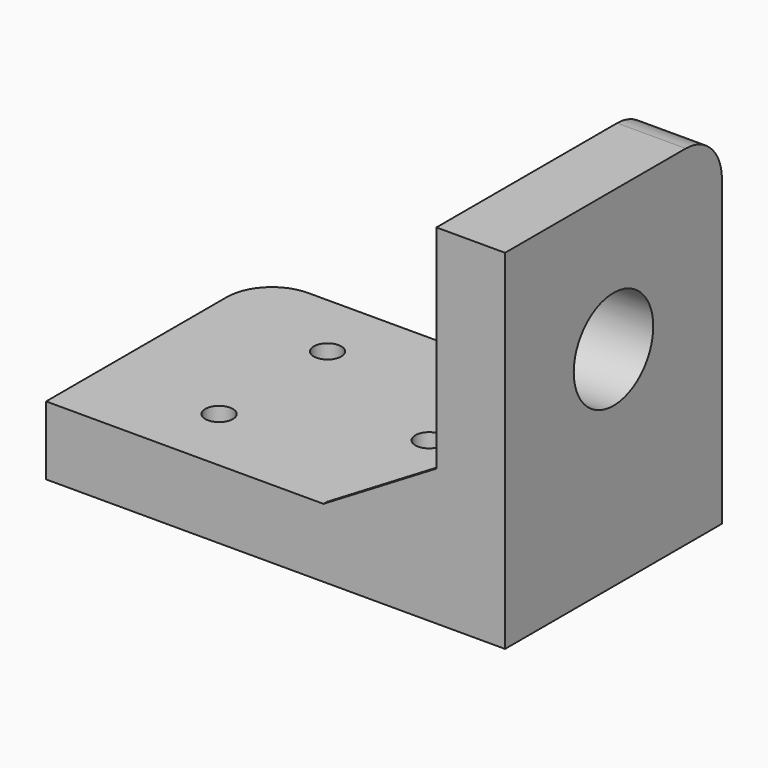
from build123d import *

# Parameters (mm, degrees)
F0_W          = 50.8
F0_H          = 30
F0_R          = 1.525
F1_DEPTH      = 7.6
F2_W          = 7.6
F2_H          = 30
F3_DEPTH      = 31
F4_R          = 5.5
F5_DEPTH      = 7.6
F6_R          = 5
F9_DEPTH      = 7
F10_DEPTH     = 7
F11_T4_DEPTH  = 48.0092585807
F11_T10_DEPTH = 48.0092585807


# Not quite as in the source:
# - a fillet or chamfer that OpenCascade refuses, or shapes differently, is made with other operations: its cross-section is extruded or revolved along the edge and cut away or added


with BuildPart() as f1:
    # F0 (on Top) → F1 (new body)
    with BuildSketch(Plane.XY):
        Rectangle(F0_W, F0_H)
        with Locations((-12.25, -7.5)):
            Circle(F0_R, mode=Mode.SUBTRACT)
        with Locations((-12.25, 7.5)):
            Circle(F0_R, mode=Mode.SUBTRACT)
        with Locations((5, 0)):
            Circle(F0_R, mode=Mode.SUBTRACT)
    extrude(amount=F1_DEPTH)

    # F2 (on face) → F3 (join)
    with BuildSketch(Plane.XY.offset(7.6)):
        with Locations((21.6, 0)):
            Rectangle(F2_W, F2_H)
    extrude(amount=F3_DEPTH)

    # F4 (on face) → F5 (cut)
    with BuildSketch(Plane(origin=(17.8, 0, 0), x_dir=(0, -1, 0), z_dir=(-1, 0, 0))):
        with Locations((0, 23.1)):
            Circle(F4_R)
    extrude(amount=-F5_DEPTH, mode=Mode.SUBTRACT)

    # F6
    f6_edges = [f1.edges().sort_by_distance(p)[0] for p in [
        (21.6, 15, 38.6),
        (-25.4, 15, 3.8),
    ]]
    fillet(f6_edges, radius=F6_R)

    # F7 (on face) → F9 (join)
    with BuildSketch(Plane(origin=(0, 15, 0), x_dir=(-1, 0, 0), z_dir=(0, 1, 0))):
        Polygon((-5.3, 7.6), (-17.8, 15.1), (-17.8, 7.6), align=None)
    extrude(amount=-F9_DEPTH)

    # F8 (on face) → F10 (join)
    with BuildSketch(Plane.XZ.offset(15)):
        Polygon((17.8, 7.6), (17.8, 15.1), (5.3, 7.6), align=None)
    extrude(amount=-F10_DEPTH)

    # F11: chamfer of 6.5 on 2 edges, made by hand


with BuildPart() as f11_tool2:
    # F11_s3 → F11_t4 (new body)
    with BuildSketch(Plane(origin=(-7.0837998008, 0, -4.2502798805), x_dir=(0, 1, 0), z_dir=(0.8574929257, 0, 0.5144957554))):
        Polygon((14.5, 3.7901187316), (8, -2.7098812684), (8, 3.7901187316), align=None)
    extrude(amount=F11_T4_DEPTH)

    split(bisect_by=Plane.YZ.offset(17.8), keep=Keep.BOTTOM)

    split(bisect_by=Plane.XY.offset(7.6), keep=Keep.TOP)


with BuildPart() as f1_1:
    add(f1.part)

    # F11_t1: cut F11_tool2
    add(f11_tool2.part, mode=Mode.SUBTRACT)


with BuildPart() as f11_tool8:
    # F11_s9 → F11_t10 (new body)
    with BuildSketch(Plane(origin=(34.0837998008, 0, 20.4502798805), x_dir=(0, 1, 0), z_dir=(-0.8574929257, 0, -0.5144957554))):
        Polygon((-8, 2.7098812684), (-14.5, -3.7901187316), (-8, -3.7901187316), align=None)
    extrude(amount=F11_T10_DEPTH)

    split(bisect_by=Plane.YZ.offset(17.8), keep=Keep.BOTTOM)

    split(bisect_by=Plane.XY.offset(7.6), keep=Keep.TOP)


with BuildPart() as f1_2:
    add(f1_1.part)

    # F11_t7: cut F11_tool8
    add(f11_tool8.part, mode=Mode.SUBTRACT)


solid = f1_2.part
